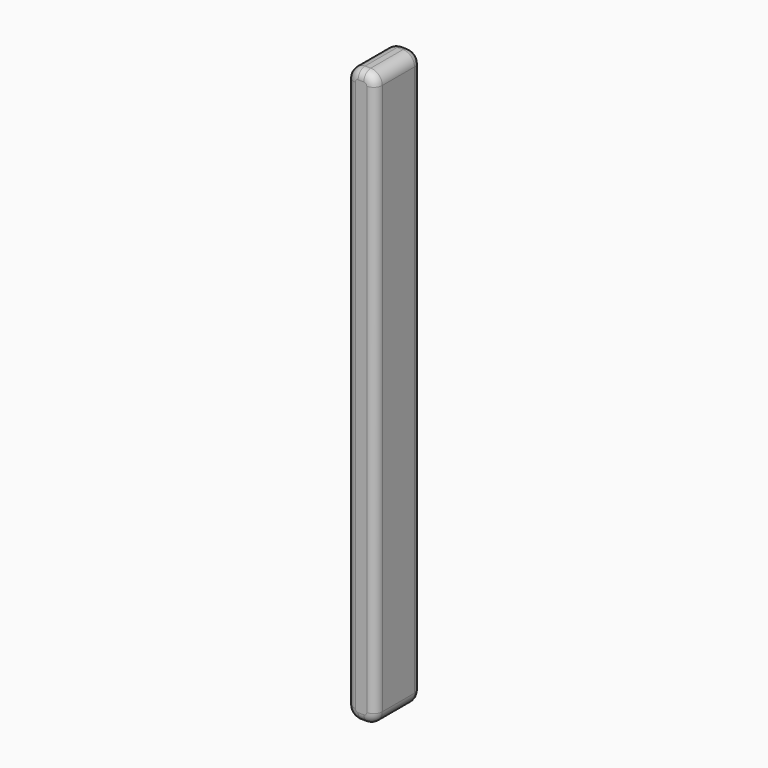
from build123d import *

# Parameters (mm, degrees)
F0_W         = 1.27
F0_H         = 25.4
F2_DEPTH     = 2.54
F3_R         = 0.381
F1_T1_DEPTH  = 2.54
F1_T4_ANGLE  = 90
F1_T6_ANGLE  = 90
F1_T8_ANGLE  = 90
F1_T10_ANGLE = 90
F1_T12_ANGLE = 90
F1_T14_ANGLE = 90
F1_T16_ANGLE = 90
F1_T18_ANGLE = 90


# Not quite as in the source:
# - a fillet or chamfer that OpenCascade refuses, or shapes differently, is made with other operations: its cross-section is extruded or revolved along the edge and cut away or added


with BuildPart() as f2:
    # F0 (on Front) → F2 (new body)
    with BuildSketch(Plane.XZ):
        with Locations((0.635, -12.7)):
            Rectangle(F0_W, F0_H)
    extrude(amount=F2_DEPTH)

    # F3
    f3_edges = [f2.edges().sort_by_distance(p)[0] for p in [
        (0.635, -2.54, 0),
        (0, -2.54, -12.7),
        (0.635, -2.54, -25.4),
        (1.27, -2.54, -12.7),
        (1.27, 0, -12.7),
        (0.635, 0, 0),
        (0, 0, -12.7),
        (0.635, 0, -25.4),
    ]]
    fillet(f3_edges, radius=F3_R)

    # F1: fillet of radius 0.508 on 4 edges, made by hand

    # F1_s2 → F1_t1 (cut)
    with BuildSketch(Plane.XZ):
        with BuildLine():
            ThreePointArc((0, -24.892), (0.1487897552, -25.2512102448), (0.508, -25.4))
            Line((0.508, -25.4), (0, -25.4))
            Line((0, -25.4), (0, -24.892))
        make_face()
        with BuildLine():
            ThreePointArc((1.27, -24.892), (1.1212102448, -25.2512102448), (0.762, -25.4))
            Line((0.762, -25.4), (1.27, -25.4))
            Line((1.27, -25.4), (1.27, -24.892))
        make_face()
        with BuildLine():
            ThreePointArc((0.508, 0), (0.1487897552, -0.1487897552), (0, -0.508))
            Line((0, -0.508), (0, 0))
            Line((0, 0), (0.508, 0))
        make_face()
        with BuildLine():
            ThreePointArc((0.762, 0), (1.1212102448, -0.1487897552), (1.27, -0.508))
            Line((1.27, -0.508), (1.27, 0))
            Line((1.27, 0), (0.762, 0))
        make_face()
    extrude(amount=F1_T1_DEPTH, mode=Mode.SUBTRACT)

    # F1_s3 → F1_t4 (revolve, cut)
    with BuildSketch(Plane.YZ.offset(0.762)):
        with BuildLine():
            ThreePointArc((0, -0.381), (-0.1115923164, -0.1115923164), (-0.381, 0))
            Line((-0.381, 0), (0, 0))
            Line((0, 0), (0, -0.381))
        make_face()
    revolve(axis=Axis((0.762, 0, -0.508), (0, 1, 0)), revolution_arc=F1_T4_ANGLE, mode=Mode.SUBTRACT)

    # F1_s5 → F1_t6 (revolve, cut)
    with BuildSketch(Plane.XY.offset(-0.508)):
        with BuildLine():
            ThreePointArc((0.889, -2.54), (1.1584076836, -2.4284076836), (1.27, -2.159))
            Line((1.27, -2.159), (1.27, -2.54))
            Line((1.27, -2.54), (0.889, -2.54))
        make_face()
    revolve(axis=Axis((0.762, -2.54, -0.508), (0, -1, 0)), revolution_arc=F1_T6_ANGLE, mode=Mode.SUBTRACT)

    # F1_s7 → F1_t8 (revolve, cut)
    with BuildSketch(Plane.XY.offset(-0.508)):
        with BuildLine():
            ThreePointArc((0.381, 0), (0.1115923164, -0.1115923164), (0, -0.381))
            Line((0, -0.381), (0, 0))
            Line((0, 0), (0.381, 0))
        make_face()
    revolve(axis=Axis((0.508, 0, -0.508), (0, 1, 0)), revolution_arc=F1_T8_ANGLE, mode=Mode.SUBTRACT)

    # F1_s9 → F1_t10 (revolve, cut)
    with BuildSketch(Plane.YZ.offset(0.508)):
        with BuildLine():
            ThreePointArc((-2.54, -0.381), (-2.4284076836, -0.1115923164), (-2.159, 0))
            Line((-2.159, 0), (-2.54, 0))
            Line((-2.54, 0), (-2.54, -0.381))
        make_face()
    revolve(axis=Axis((0.508, -2.54, -0.508), (0, -1, 0)), revolution_arc=F1_T10_ANGLE, mode=Mode.SUBTRACT)

    # F1_s11 → F1_t12 (revolve, cut)
    with BuildSketch(Plane.XY.offset(-24.892)):
        with BuildLine():
            ThreePointArc((0.889, 0), (1.1584076836, -0.1115923164), (1.27, -0.381))
            Line((1.27, -0.381), (1.27, 0))
            Line((1.27, 0), (0.889, 0))
        make_face()
    revolve(axis=Axis((0.762, 0, -24.892), (0, 1, 0)), revolution_arc=F1_T12_ANGLE, mode=Mode.SUBTRACT)

    # F1_s13 → F1_t14 (revolve, cut)
    with BuildSketch(Plane.YZ.offset(0.762)):
        with BuildLine():
            ThreePointArc((-2.54, -25.019), (-2.4284076836, -25.2884076836), (-2.159, -25.4))
            Line((-2.159, -25.4), (-2.54, -25.4))
            Line((-2.54, -25.4), (-2.54, -25.019))
        make_face()
    revolve(axis=Axis((0.762, -2.54, -24.892), (0, -1, 0)), revolution_arc=F1_T14_ANGLE, mode=Mode.SUBTRACT)

    # F1_s15 → F1_t16 (revolve, cut)
    with BuildSketch(Plane.YZ.offset(0.508)):
        with BuildLine():
            ThreePointArc((0, -25.019), (-0.1115923164, -25.2884076836), (-0.381, -25.4))
            Line((-0.381, -25.4), (0, -25.4))
            Line((0, -25.4), (0, -25.019))
        make_face()
    revolve(axis=Axis((0.508, 0, -24.892), (0, 1, 0)), revolution_arc=F1_T16_ANGLE, mode=Mode.SUBTRACT)

    # F1_s17 → F1_t18 (revolve, cut)
    with BuildSketch(Plane.XY.offset(-24.892)):
        with BuildLine():
            ThreePointArc((0.381, -2.54), (0.1115923164, -2.4284076836), (0, -2.159))
            Line((0, -2.159), (0, -2.54))
            Line((0, -2.54), (0.381, -2.54))
        make_face()
    revolve(axis=Axis((0.508, -2.54, -24.892), (0, -1, 0)), revolution_arc=F1_T18_ANGLE, mode=Mode.SUBTRACT)


solid = f2.part
